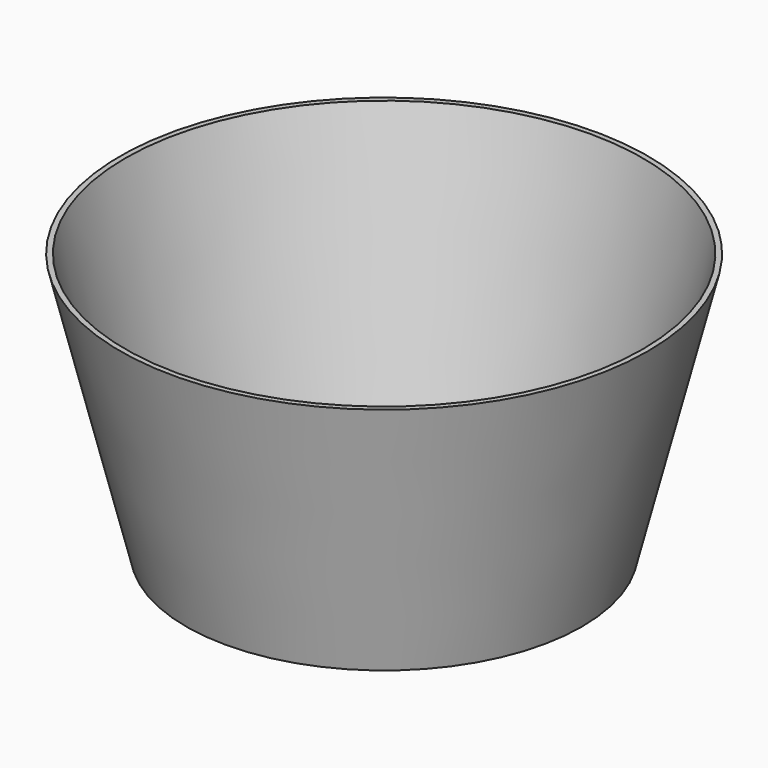
from build123d import *

# Parameters (mm, degrees)
F0_R     = 20
F1_DEPTH = 20
F2_SIZE2 = 4.99999
F2_SIZE  = 19.99999
F3_R     = 19.6
F4_DEPTH = 19
F4_TAPER = 14


# Not quite as in the source:
# - a fillet or chamfer is up to 0.001 mm smaller than in the source, because OpenCascade refuses the exact size


with BuildPart() as f1:
    # F0 (on Top) → F1 (new body)
    with BuildSketch(Plane.XY):
        Circle(F0_R)
    extrude(amount=F1_DEPTH)

    # F2 (size 20 and 5 in the source; OpenCascade refuses exactly that, so slightly less here)
    f2_edges = [f1.edges().sort_by_distance(p)[0] for p in [
        (-20, 0, 0),
    ]]
    f2_side = f1.faces().sort_by_distance((-20, 0, 10))[0]
    chamfer(f2_edges, length=F2_SIZE, length2=F2_SIZE2, reference=f2_side)

    # F3 (on face) → F4 (cut)
    with BuildSketch(Plane.XY.offset(20)):
        Circle(F3_R)
    extrude(amount=-F4_DEPTH, taper=F4_TAPER, mode=Mode.SUBTRACT)


solid = f1.part
